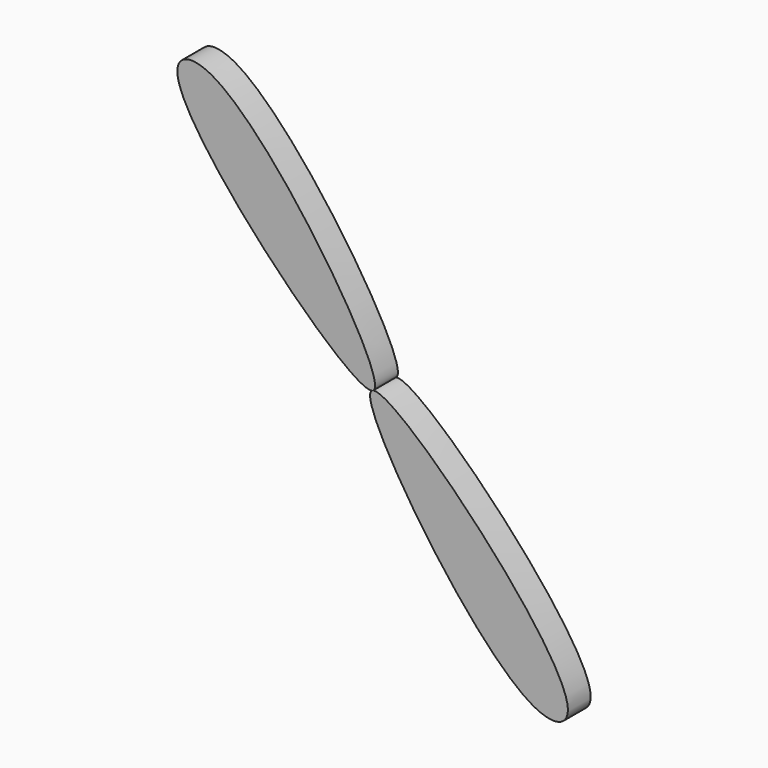
from build123d import *

# Parameters (mm, degrees)
F1_DEPTH = 12.7


# Not quite as in the source:
# - ends of sketch curves that miss each other by under 0.0002 mm in the source are joined


with BuildPart() as f1:
    # F0 (on Front) → F1 (new body)
    with BuildSketch(Plane.XZ):
        with BuildLine():
            add(Edge.make_bspline(
                [(0.057148097, 0.0244964621), (9.83409264, 3.651025559), (107.92779337, -96.0539163979), (62.01166785, -113.0410639025), (-9.0442422082, -4.4336636114), (-0.0968406225, -0.0415107744)],
                knots=[0.0023124215, 0.0023124215, 0.0023124215, 0.0023124215, 0.4274724605, 0.581813776, 1, 1, 1, 1], degree=3))
            add(Edge.make_bspline(
                [(0.057148097, 0.0244964621), (0.0076722315, 0.0002091649), (-0.0436642788, -0.0217865361), (-0.0968406225, -0.0415107744)],
                knots=[0, 0, 0, 0, 0.0023124215, 0.0023124215, 0.0023124215, 0.0023124215], degree=3))
        make_face()
        with BuildLine():
            add(Edge.make_bspline(
                [(-0.0968406225, -0.0415107744), (-0.0473646645, -0.0172237267), (0.0039718458, 0.0047719743), (0.057148097, 0.0244964621)],
                knots=[0, 0, 0, 0, 0.0023124215, 0.0023124215, 0.0023124215, 0.0023124215], degree=3))
            add(Edge.make_bspline(
                [(-0.0968406225, -0.0415107744), (-9.873785171, -3.6680401433), (-107.9674864943, 96.0369021462), (-62.0513603609, 113.0240496125), (9.0045498695, 4.4166490622), (0.057148097, 0.0244964621)],
                knots=[0.0023124215, 0.0023124215, 0.0023124215, 0.0023124215, 0.4274724602, 0.5818137766, 1, 1, 1, 1], degree=3))
        make_face()
        with BuildLine():
            add(Edge.make_bspline(
                [(0.0571481896, 0.0244962124), (0.0076722315, 0.0002091649), (-0.0436642788, -0.0217865361), (-0.0968405301, -0.0415110237)],
                knots=[0, 0, 0, 0, 0.0023124215, 0.0023124215, 0.0023124215, 0.0023124215], degree=3))
            add(Edge.make_bspline(
                [(-0.0968405301, -0.0415110237), (-0.0473646645, -0.0172237267), (0.0039718458, 0.0047719743), (0.0571481896, 0.0244962124)],
                knots=[0, 0, 0, 0, 0.0023124215, 0.0023124215, 0.0023124215, 0.0023124215], degree=3))
        make_face()
    extrude(amount=F1_DEPTH)


solid = f1.part
